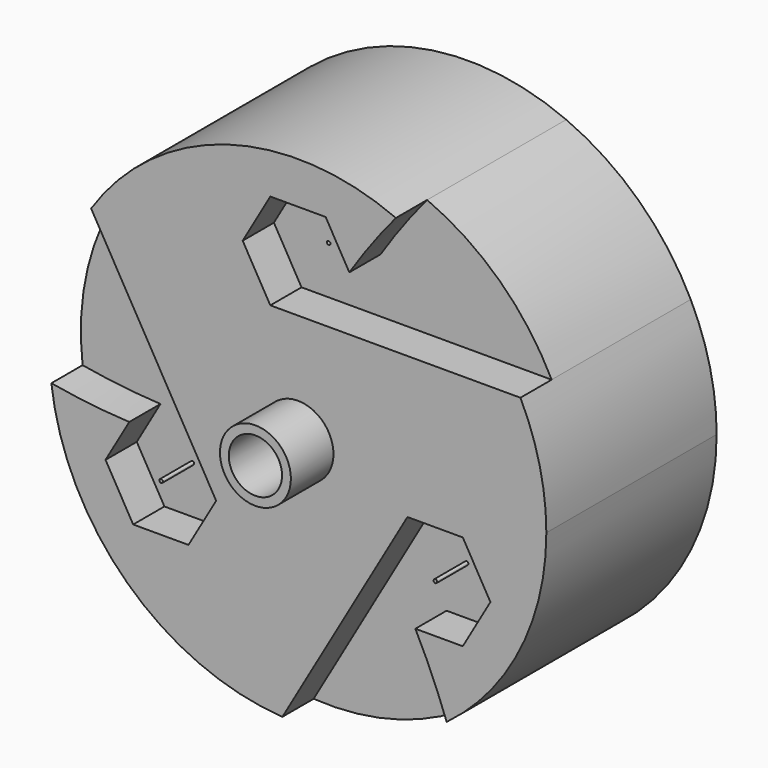
from build123d import *

# Parameters (mm, degrees)
F0_R      = 2
F0_R_2    = 0.1
F1_DEPTH  = 12
F0_R_3    = 1.5
F2_DEPTH  = 15
F4_R      = 0.1
F5_DEPTH  = 2
F6_COUNT  = 3
F5_FACE_R = 0.1
F6_FACE_R = 0.1
F7_DEPTH  = 4.2


# Not quite as in the source:
# - a fillet or chamfer that OpenCascade refuses, or shapes differently, is made with other operations: its cross-section is extruded or revolved along the edge and cut away or added


with BuildPart() as f1:
    # F0 (on Front) → F1 (new body)
    with BuildSketch(Plane.XZ):
        with BuildLine():
            ThreePointArc((4.7997142496, 7.1366126269), (-12.410762485, -13.4329699503), (13.278817402, -5.728833265))
            ThreePointArc((13.278817402, -5.728833265), (12.9087772386, -2.5313037732), (11.8182181375, 0.4971950993))
            Line((11.8182181375, 0.4971950993), (-2.2800283653, 0.4971950993))
            Line((-2.2800283653, 0.4971950993), (-3.8388741325, 3.1971951693))
            Line((-3.8388741325, 3.1971951693), (-2.2800283653, 5.8971952394))
            Line((-2.2800283653, 5.8971952394), (0.8376631692, 5.8971952394))
            Line((0.8376631692, 5.8971952394), (2.174251278, 3.5821567261))
            ThreePointArc((2.174251278, 3.5821567261), (3.4311500139, 5.4006249736), (4.7997142496, 7.1366126269))
        make_face()
        with Locations((-0.721182598, -5.728833265)):
            Circle(F0_R, mode=Mode.SUBTRACT)
        with BuildLine():
            Line((-2.2800283653, 0.4971950993), (11.8182181375, 0.4971950993))
            ThreePointArc((11.8182181375, 0.4971950993), (8.8998388381, 4.4415131659), (4.7997142496, 7.1366126269))
            ThreePointArc((4.7997142496, 7.1366126269), (3.4311500139, 5.4006249736), (2.174251278, 3.5821567261))
            Line((2.174251278, 3.5821567261), (0.8376631692, 5.8971952394))
            Line((0.8376631692, 5.8971952394), (-2.2800283653, 5.8971952394))
            Line((-2.2800283653, 5.8971952394), (-3.8388741325, 3.1971951693))
            Line((-3.8388741325, 3.1971951693), (-2.2800283653, 0.4971950993))
        make_face()
        with Locations((-0.7538866513, 3.197135257)):
            Circle(F0_R_2, mode=Mode.SUBTRACT)
    extrude(amount=F1_DEPTH)

    # F0 (on Front) → F2 (join)
    with BuildSketch(Plane.XZ):
        with Locations((-0.721182598, -5.728833265)):
            Circle(F0_R)
        with Locations((-0.721182598, -5.728833265)):
            Circle(F0_R_3, mode=Mode.SUBTRACT)
    extrude(amount=F2_DEPTH)

    # F3: chamfer of 9 x 11.5194746897 on 1 edges, made by hand

    # F3_s1 → F3_t2 (revolve, cut)
    with BuildSketch(Plane.XY.offset(-5.728833265)):
        Polygon((12.2982920917, 0), (0.778817402, -9), (0.778817402, 0), align=None)
    revolve(axis=Axis((-0.721182598, 0, -5.728833265), (0, -1, 0)), mode=Mode.SUBTRACT)

    # F6: F5 ×3 about axis
    f6_axis = Axis((-0.721182598, 0, -5.728833265), (0, -1, 0))


with BuildPart() as f5:
    # F4 (on face) → F5 (new body)
    with BuildSketch(Plane.XZ.offset(12)):
        with BuildLine():
            Line((-2.2800283653, 0.4971950993), (11.8182181375, 0.4971950993))
            ThreePointArc((11.8182181375, 0.4971950993), (8.8998388381, 4.4415131659), (4.7997142496, 7.1366126269))
            ThreePointArc((4.7997142496, 7.1366126269), (3.4311500139, 5.4006249736), (2.174251278, 3.5821567261))
            Line((2.174251278, 3.5821567261), (0.8376631692, 5.8971952394))
            Line((0.8376631692, 5.8971952394), (-2.2800283653, 5.8971952394))
            Line((-2.2800283653, 5.8971952394), (-3.8388741325, 3.1971951693))
            Line((-3.8388741325, 3.1971951693), (-2.2800283653, 0.4971950993))
        make_face()
        with Locations((-0.7538866513, 3.197135257)):
            Circle(F4_R, mode=Mode.SUBTRACT)
    extrude(amount=F5_DEPTH)


with BuildPart() as f1_1:
    add(f1.part)
    for i in range(1, F6_COUNT):
        add(f5.part.rotate(f6_axis, i * 360 / F6_COUNT))


with BuildPart() as f7_tool:
    # F5_face (on face) + F6_face (on face) → F7 (new body)
    with BuildSketch(Plane(origin=(3.5829132763, -14, 3.0354703716), x_dir=(1, 0, 0), z_dir=(0, -1, 0))):
        with BuildLine():
            Line((-5.8629416416, 2.8617248677), (-7.4217874088, 0.1617247977))
            Line((-7.4217874088, 0.1617247977), (-5.8629416416, -2.5382752723))
            Line((-5.8629416416, -2.5382752723), (8.2353048612, -2.5382752723))
            ThreePointArc((8.2353048612, -2.5382752723), (5.3169255618, 1.4060427943), (1.2168009733, 4.1011422553))
            ThreePointArc((1.2168009733, 4.1011422553), (-0.1517632624, 2.365154602), (-1.4086619983, 0.5466863545))
            Line((-1.4086619983, 0.5466863545), (-2.7452501071, 2.8617248677))
            Line((-2.7452501071, 2.8617248677), (-5.8629416416, 2.8617248677))
        make_face()
        with Locations((-4.3367999276, 0.1616648853)):
            Circle(F5_FACE_R, mode=Mode.SUBTRACT)
    with BuildSketch(Plane(origin=(4.7168790606, -14, -13.8384414508), x_dir=(1, 0, 0), z_dir=(0, -1, 0))):
        with BuildLine():
            Line((5.4097972549, 3.6465939687), (3.8509514876, 6.3465940387))
            Line((3.8509514876, 6.3465940387), (0.7332599531, 6.3465940387))
            Line((0.7332599531, 6.3465940387), (-6.3158632983, -5.8628455816))
            ThreePointArc((-6.3158632983, -5.8628455816), (-1.4407940022, -5.3076140037), (2.943292891, -3.1043516819))
            ThreePointArc((2.943292891, -3.1043516819), (2.1241656004, -1.0511464604), (1.17777527, 0.9465938986))
            Line((1.17777527, 0.9465938986), (3.8509514876, 0.9465938986))
            Line((3.8509514876, 0.9465938986), (5.4097972549, 3.6465939687))
        make_face()
        with Locations((2.3084058614, 3.6749464658)):
            Circle(F6_FACE_R, mode=Mode.SUBTRACT)
        with BuildLine():
            Line((-14.7270748049, 0.9465938986), (-11.6093832704, 0.9465938986))
            Line((-11.6093832704, 0.9465938986), (-10.0505375032, 3.6465939687))
            Line((-10.0505375032, 3.6465939687), (-17.0996607546, 15.8560335889))
            ThreePointArc((-17.0996607546, 15.8560335889), (-19.0563507512, 11.3564839444), (-19.3403130559, 6.4581221616))
            ThreePointArc((-19.3403130559, 6.4581221616), (-17.1526215296, 6.1409045934), (-14.9493324633, 5.9616324819))
            Line((-14.9493324633, 5.9616324819), (-16.2859205721, 3.6465939687))
            Line((-16.2859205721, 3.6465939687), (-14.7270748049, 0.9465938986))
        make_face()
        with Locations((-13.1518251254, 3.6183013839)):
            Circle(F6_FACE_R, mode=Mode.SUBTRACT)
    extrude(amount=-F7_DEPTH)


with BuildPart() as f1_2:
    add(f1_1.part)

    # F7: cut by f7_tool
    add(f7_tool.part, mode=Mode.SUBTRACT)


with BuildPart() as f5_1:
    add(f5.part)

    # F7: cut by f7_tool
    add(f7_tool.part, mode=Mode.SUBTRACT)


solid = f1_2.part
